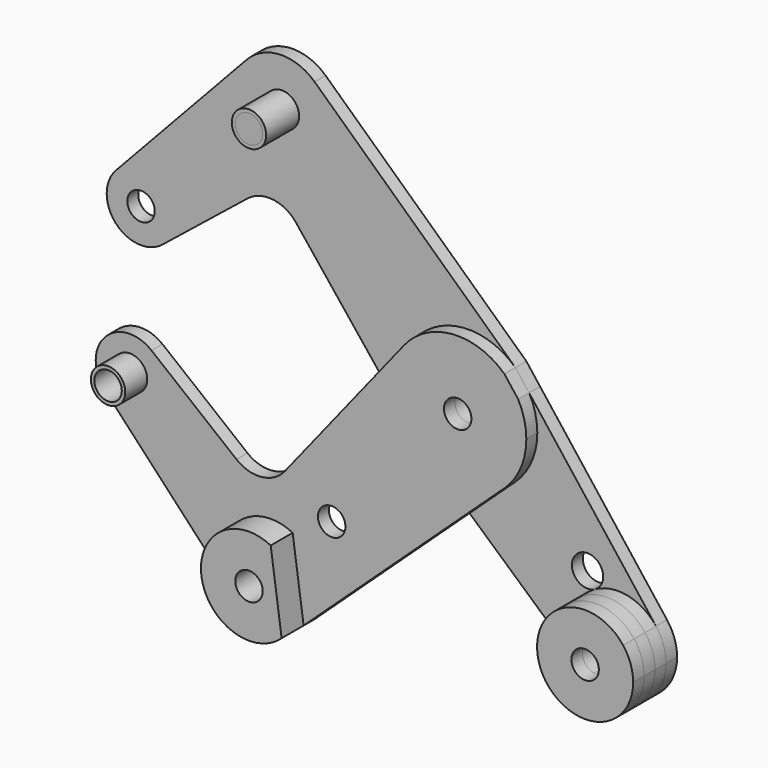
from build123d import *

# Parameters (mm, degrees)
F0_R     = 3.175
F0_R_2   = 3.9751
F1_DEPTH = 3.175
F2_DEPTH = 3.175
F4_R     = 3.175
F6_DEPTH = 6.35
F4_R_2   = 3.9751
F3_R     = 3.9751
F3_R_2   = 3.175


# Not quite as in the source:
# - a pattern or mirror of a feature is missing from the dataset's text; its kind, count and spacing are read off the source's solid


with BuildPart() as f1:
    # F0 (on Front) → F1 (new body)
    with BuildSketch(Plane.XZ):
        with BuildLine():
            ThreePointArc((-12.4155922988, 9.8928607021), (-1.190625, 15.8302885984), (10.7961672163, 11.6386596495))
            Line((10.7961672163, 11.6386596495), (-35.6273518138, 54.7017003528))
            ThreePointArc((-35.6273518138, 54.7017003528), (-32.9996715166, 50.9991279116), (-32.0721688652, 46.5546385981))
            ThreePointArc((-32.0721688652, 46.5546385981), (-47.2623367435, 36.2173139479), (-51.3046153758, 54.141082094))
            Line((-51.3046153758, 54.141082094), (-81.5728776771, 21.7442586038))
            ThreePointArc((-81.5728776771, 21.7442586038), (-72.8602959708, 23.709173714), (-67.8354158839, 16.3253703924))
            ThreePointArc((-67.8354158839, 16.3253703924), (-68.6160171621, 12.8927756107), (-70.8042869228, 10.1353273799))
            Line((-70.8042869228, 10.1353273799), (-51.1479269508, 25.9131110286))
            ThreePointArc((-51.1479269508, 25.9131110286), (-45.2921470677, 27.6145996041), (-39.9536195601, 24.6675085869))
            Line((-39.9536195601, 24.6675085869), (-20.2983167404, 0))
            Line((-20.2983167404, 0), (-12.4155922988, 9.8928607021))
        make_face()
        with BuildLine():
            ThreePointArc((-67.8354158839, 16.3253703924), (-72.8602959708, 23.709173714), (-81.5728776771, 21.7442586038))
            ThreePointArc((-81.5728776771, 21.7442586038), (-81.5922457087, 10.9272867843), (-70.8042869228, 10.1353273799))
            ThreePointArc((-70.8042869228, 10.1353273799), (-68.6160171621, 12.8927756107), (-67.8354158839, 16.3253703924))
        make_face()
        with Locations((-75.7729158839, 16.3253703924)):
            Circle(F0_R, mode=Mode.SUBTRACT)
        with BuildLine():
            ThreePointArc((-32.0721688652, 46.5546385981), (-32.9996715166, 50.9991279116), (-35.6273518138, 54.7017003528))
            ThreePointArc((-35.6273518138, 54.7017003528), (-43.581797541, 57.6600402147), (-51.3046153758, 54.141082094))
            ThreePointArc((-51.3046153758, 54.141082094), (-47.2623367435, 36.2173139479), (-32.0721688652, 46.5546385981))
        make_face()
        with Locations((-43.1846688652, 46.5546385981)):
            Circle(F0_R, mode=Mode.SUBTRACT)
        with BuildLine():
            Line((43.3386214046, -30.4460661325), (13.9807141591, 7.5203229054))
            ThreePointArc((13.9807141591, 7.5203229054), (15.3941460022, 3.8776144551), (15.875, 0))
            ThreePointArc((15.875, 0), (14.5499962124, -6.3492704479), (10.7961672163, -11.6386596495))
            Line((10.7961672163, -11.6386596495), (0.2019726407, -21.4659679139))
            Line((0.2019726407, -21.4659679139), (27.1450533438, -45.5315308079))
            ThreePointArc((27.1450533438, -45.5315308079), (23.5080187906, -35.9739391549), (29.2199730699, -27.4916542706))
            ThreePointArc((29.2199730699, -27.4916542706), (36.8237941478, -26.366799027), (43.3386214046, -30.4460661325))
        make_face()
        with BuildLine():
            ThreePointArc((31.1003708361, -24.3216324516), (30.5949064185, -26.1645197306), (29.2199730699, -27.4916542706))
            ThreePointArc((29.2199730699, -27.4916542706), (24.3813350251, -22.4787451727), (31.1003708361, -24.3216324516))
        make_face(mode=Mode.SUBTRACT)
        with BuildLine():
            Line((13.9807141591, 7.5203229054), (10.7961672163, 11.6386596495))
            ThreePointArc((10.7961672163, 11.6386596495), (-1.190625, 15.8302885984), (-12.4155922988, 9.8928607021))
            ThreePointArc((-12.4155922988, 9.8928607021), (-15.875, 0), (-12.4155922988, -9.8928607021))
            ThreePointArc((-12.4155922988, -9.8928607021), (-11.5365681923, -10.9051923112), (-10.5752596405, -11.8397427563))
            ThreePointArc((-10.5752596405, -11.8397427563), (0.1493607821, -15.87429735), (10.7961672163, -11.6386596495))
            ThreePointArc((10.7961672163, -11.6386596495), (14.5499962124, -6.3492704479), (15.875, 0))
            ThreePointArc((15.875, 0), (15.3941460022, 3.8776144551), (13.9807141591, 7.5203229054))
        make_face()
        Circle(F0_R_2, mode=Mode.SUBTRACT)
        with BuildLine():
            ThreePointArc((45.6602350922, -37.2437108785), (45.0638270563, -33.6521282118), (43.3386214046, -30.4460661325))
            ThreePointArc((43.3386214046, -30.4460661325), (36.8237941478, -26.366799027), (29.2199730699, -27.4916542706))
            ThreePointArc((29.2199730699, -27.4916542706), (23.5080187906, -35.9739391549), (27.1450533438, -45.5315308079))
            ThreePointArc((27.1450533438, -45.5315308079), (39.0878537757, -47.3864412106), (45.6602350922, -37.2437108785))
        make_face()
        with Locations((34.5477350922, -37.2437108785)):
            Circle(F0_R, mode=Mode.SUBTRACT)
        with BuildLine():
            ThreePointArc((-12.4155922988, -9.8928607021), (-15.875, 0), (-12.4155922988, 9.8928607021))
            Line((-12.4155922988, 9.8928607021), (-20.2983167404, 0))
            Line((-20.2983167404, 0), (-12.4155922988, -9.8928607021))
        make_face()
        with BuildLine():
            ThreePointArc((10.7961672163, -11.6386596495), (0.1493607821, -15.87429735), (-10.5752596405, -11.8397427563))
            Line((-10.5752596405, -11.8397427563), (0.2019726407, -21.4659679139))
            Line((0.2019726407, -21.4659679139), (10.7961672163, -11.6386596495))
        make_face()
        Circle(F0_R_2)
        Circle(F0_R, mode=Mode.SUBTRACT)
    extrude(amount=-F1_DEPTH)


with BuildPart() as f2:
    # F0 (on Front) → F2 (new body)
    with BuildSketch(Plane.XZ):
        with BuildLine():
            ThreePointArc((-10.5752596405, -11.8397427563), (-11.5365681923, -10.9051923112), (-12.4155922988, -9.8928607021))
            Line((-12.4155922988, -9.8928607021), (-20.2983167404, 0))
            Line((-20.2983167404, 0), (-39.9536195601, -24.6675085869))
            ThreePointArc((-39.9536195601, -24.6675085869), (-45.2921470677, -27.6145996041), (-51.1479269508, -25.9131110286))
            Line((-51.1479269508, -25.9131110286), (-70.8042869228, -10.1353273799))
            ThreePointArc((-70.8042869228, -10.1353273799), (-68.6160171621, -12.8927756107), (-67.8354158839, -16.3253703924))
            ThreePointArc((-67.8354158839, -16.3253703924), (-72.8602959708, -23.709173714), (-81.5728776771, -21.7442586038))
            Line((-81.5728776771, -21.7442586038), (-51.3046153758, -54.141082094))
            ThreePointArc((-51.3046153758, -54.141082094), (-47.2623367435, -36.2173139479), (-32.0721688652, -46.5546385981))
            ThreePointArc((-32.0721688652, -46.5546385981), (-32.9996715166, -50.9991279116), (-35.6273518138, -54.7017003528))
            Line((-35.6273518138, -54.7017003528), (0.2019726407, -21.4659679139))
            Line((0.2019726407, -21.4659679139), (-10.5752596405, -11.8397427563))
        make_face()
        with Locations((-29.1410145503, -31.415070126)):
            Circle(F0_R, mode=Mode.SUBTRACT)
        with BuildLine():
            ThreePointArc((-67.8354158839, -16.3253703924), (-68.6160171621, -12.8927756107), (-70.8042869228, -10.1353273799))
            ThreePointArc((-70.8042869228, -10.1353273799), (-81.5922457087, -10.9272867843), (-81.5728776771, -21.7442586038))
            ThreePointArc((-81.5728776771, -21.7442586038), (-72.8602959708, -23.709173714), (-67.8354158839, -16.3253703924))
        make_face()
        with Locations((-75.7729158839, -16.3253703924)):
            Circle(F0_R, mode=Mode.SUBTRACT)
        with BuildLine():
            ThreePointArc((-51.3046153758, -54.141082094), (-43.581797541, -57.6600402147), (-35.6273518138, -54.7017003528))
            ThreePointArc((-35.6273518138, -54.7017003528), (-32.9996715166, -50.9991279116), (-32.0721688652, -46.5546385981))
            ThreePointArc((-32.0721688652, -46.5546385981), (-47.2623367435, -36.2173139479), (-51.3046153758, -54.141082094))
        make_face()
        with Locations((-43.1846688652, -46.5546385981)):
            Circle(F0_R, mode=Mode.SUBTRACT)
        with BuildLine():
            ThreePointArc((-12.4155922988, -9.8928607021), (-15.875, 0), (-12.4155922988, 9.8928607021))
            Line((-12.4155922988, 9.8928607021), (-20.2983167404, 0))
            Line((-20.2983167404, 0), (-12.4155922988, -9.8928607021))
        make_face()
        with BuildLine():
            Line((13.9807141591, 7.5203229054), (10.7961672163, 11.6386596495))
            ThreePointArc((10.7961672163, 11.6386596495), (-1.190625, 15.8302885984), (-12.4155922988, 9.8928607021))
            ThreePointArc((-12.4155922988, 9.8928607021), (-15.875, 0), (-12.4155922988, -9.8928607021))
            ThreePointArc((-12.4155922988, -9.8928607021), (-11.5365681923, -10.9051923112), (-10.5752596405, -11.8397427563))
            ThreePointArc((-10.5752596405, -11.8397427563), (0.1493607821, -15.87429735), (10.7961672163, -11.6386596495))
            ThreePointArc((10.7961672163, -11.6386596495), (14.5499962124, -6.3492704479), (15.875, 0))
            ThreePointArc((15.875, 0), (15.3941460022, 3.8776144551), (13.9807141591, 7.5203229054))
        make_face()
        Circle(F0_R_2, mode=Mode.SUBTRACT)
        with BuildLine():
            ThreePointArc((10.7961672163, -11.6386596495), (0.1493607821, -15.87429735), (-10.5752596405, -11.8397427563))
            Line((-10.5752596405, -11.8397427563), (0.2019726407, -21.4659679139))
            Line((0.2019726407, -21.4659679139), (10.7961672163, -11.6386596495))
        make_face()
        Circle(F0_R_2)
        Circle(F0_R, mode=Mode.SUBTRACT)
    extrude(amount=F2_DEPTH)


with BuildPart() as f6:
    # F4 (on face) → F6 (new body, through all)
    with BuildSketch(Plane.XZ.offset(3.175)):
        with BuildLine():
            Line((-35.6273518138, -54.7017003528), (-38.1655655345, -36.6401916642))
            ThreePointArc((-38.1655655345, -36.6401916642), (-52.0714060936, -39.882790452), (-51.3046153758, -54.141082094))
            ThreePointArc((-51.3046153758, -54.141082094), (-43.581797541, -57.6600402147), (-35.6273518138, -54.7017003528))
        make_face()
        with Locations((-43.1846688652, -46.5546385981)):
            Circle(F4_R, mode=Mode.SUBTRACT)
    extrude(amount=F6_DEPTH)


with BuildPart() as f6b:
    # F4 (on face) → F6, piece 2 (new body, through all)
    with BuildSketch(Plane.XZ.offset(3.175)):
        with Locations((-75.7729158839, -16.3253703924)):
            Circle(F4_R_2)
        with Locations((-75.7729158839, -16.3253703924)):
            Circle(F4_R, mode=Mode.SUBTRACT)
    extrude(amount=F6_DEPTH)


with BuildPart() as f6c:
    # F0 (on Front) → F6, piece 3 (new body, through all)
    with BuildSketch(Plane.XZ):
        with BuildLine():
            ThreePointArc((45.6602350922, -37.2437108785), (45.0638270563, -33.6521282118), (43.3386214046, -30.4460661325))
            ThreePointArc((43.3386214046, -30.4460661325), (36.8237941478, -26.366799027), (29.2199730699, -27.4916542706))
            ThreePointArc((29.2199730699, -27.4916542706), (23.5080187906, -35.9739391549), (27.1450533438, -45.5315308079))
            ThreePointArc((27.1450533438, -45.5315308079), (39.0878537757, -47.3864412106), (45.6602350922, -37.2437108785))
        make_face()
        with Locations((34.5477350922, -37.2437108785)):
            Circle(F0_R, mode=Mode.SUBTRACT)
    extrude(amount=F6_DEPTH)

    # F6_3_copies: F6c across plane


with BuildPart() as f6d:
    # F0 (on Front) → F6, piece 4 (new body, through all)
    with BuildSketch(Plane.XZ):
        with Locations((-43.1846688652, 46.5546385981)):
            Circle(F0_R)
    extrude(amount=F6_DEPTH)

    # F6_4_copies: F6d across plane


with BuildPart() as f6e:
    # F3 (on face) → F6, piece 5 (new body, through all)
    with BuildSketch(Plane.XZ):
        with Locations((-43.1846688652, 46.5546385981)):
            Circle(F3_R)
        with Locations((-43.1846688652, 46.5546385981)):
            Circle(F3_R_2, mode=Mode.SUBTRACT)
    extrude(amount=F6_DEPTH)

    # F6_5_copies: F6e across plane


with BuildPart() as f6c_1:
    add(f6c.part)
    add(f6c.part.mirror(Plane(origin=(0, -4.7625, 0), x_dir=(0, 0, -1), z_dir=(0, -1, 0))))


with BuildPart() as f6d_1:
    add(f6d.part)
    add(f6d.part.mirror(Plane(origin=(0, -4.7625, 0), x_dir=(0, 0, -1), z_dir=(0, -1, 0))))


with BuildPart() as f6e_1:
    add(f6e.part)
    add(f6e.part.mirror(Plane(origin=(0, -4.7625, 0), x_dir=(0, 0, -1), z_dir=(0, -1, 0))))


solid = Compound([f1.part, f2.part, f6.part, f6b.part, f6c_1.part, f6d_1.part, f6e_1.part])
